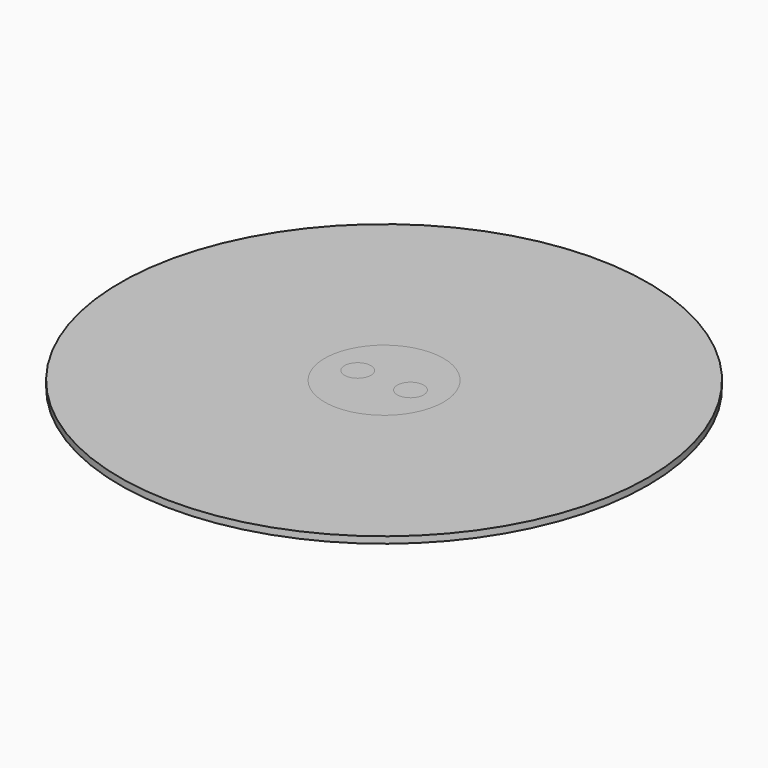
from build123d import *

# Parameters (mm, degrees)
F0_R      = 20
F1_DEPTH  = 0.5
F2_R      = 5
F3_DEPTH  = 5
F4_R      = 4.5
F5_DEPTH  = 25
F6_R      = 4.5
F7_DEPTH  = 5
F8_R      = 1
F9_DEPTH  = 8
F11_DEPTH = 3
F12_R     = 1
F13_DEPTH = 25


with BuildPart() as f1:
    # F0 (on Top) → F1 (new body)
    with BuildSketch(Plane.XY):
        Circle(F0_R)
    extrude(amount=F1_DEPTH)

    # F2 (on face) → F3 (join)
    with BuildSketch(Plane.XY.offset(0.5)):
        Circle(F2_R)
    extrude(amount=-F3_DEPTH)

    # F4 (on face) → F5 (cut)
    with BuildSketch(Plane.XY.offset(0.5)):
        Circle(F4_R)
    extrude(amount=-F5_DEPTH, mode=Mode.SUBTRACT)


with BuildPart() as f7:
    # F6 (on face) → F7 (new body)
    with BuildSketch(Plane.XY.offset(0.5)):
        Circle(F6_R)
    extrude(amount=-F7_DEPTH)

    # F12 (on face) → F13 (cut)
    with BuildSketch(Plane.XY.offset(0.5)):
        with Locations((-2, 0)):
            Circle(F12_R)
        with Locations((2, 0)):
            Circle(F12_R)
    extrude(amount=-F13_DEPTH, mode=Mode.SUBTRACT)


with BuildPart() as f9:
    # F8 (on face) → F9 (new body)
    with BuildSketch(Plane.XY.offset(0.5)):
        with Locations((-2, 0)):
            Circle(F8_R)
    extrude(amount=-F9_DEPTH)


with BuildPart() as f9b:
    # F8 (on face) → F9, piece 2 (new body)
    with BuildSketch(Plane.XY.offset(0.5)):
        with Locations((2, 0)):
            Circle(F8_R)
    extrude(amount=-F9_DEPTH)


with BuildPart() as f11_tool:
    # F10 (on face) → F11 (new body)
    with BuildSketch(Plane(origin=(0, 0, -7.5), x_dir=(1, 0, 0), z_dir=(0, 0, -1))):
        with BuildLine():
            Line((-1.25, 0), (-1, 0))
            ThreePointArc((-1, 0), (-2, 1), (-3, 0))
            Line((-3, 0), (-2.75, 0))
            ThreePointArc((-2.75, 0), (-2, -0.75), (-1.25, 0))
        make_face()
        with BuildLine():
            Line((2.75, 0), (3, 0))
            ThreePointArc((3, 0), (2, 1), (1, 0))
            Line((1, 0), (1.25, 0))
            ThreePointArc((1.25, 0), (2, -0.75), (2.75, 0))
        make_face()
    extrude(amount=-F11_DEPTH)


with BuildPart() as f9_1:
    add(f9.part)

    # F11: cut by f11_tool
    add(f11_tool.part, mode=Mode.SUBTRACT)


with BuildPart() as f9b_1:
    add(f9b.part)

    # F11: cut by f11_tool
    add(f11_tool.part, mode=Mode.SUBTRACT)


solid = Compound([f1.part, f7.part, f9_1.part, f9b_1.part])
